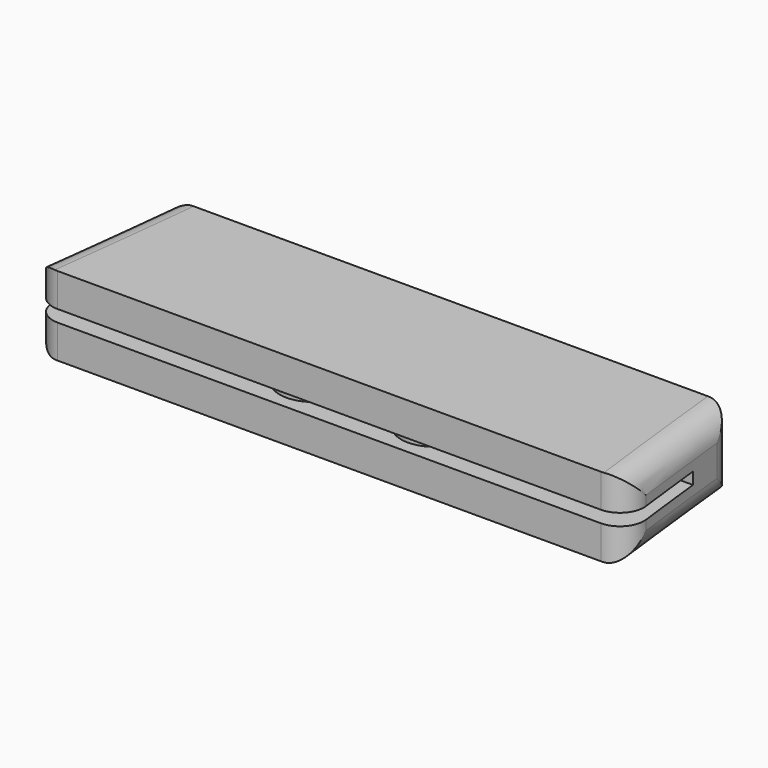
from build123d import *

# Parameters (mm, degrees)
F1_DEPTH = 4.191
F2_W     = 31.75
F2_H     = 0.635
F3_DEPTH = 5.08
F5_DEPTH = 4.191
F6_R     = 1.27


with BuildPart() as f1:
    # F0 (on Top) → F1 (new body)
    with BuildSketch(Plane.XY):
        with BuildLine():
            Line((30.8222222764, 8.072550722), (0.9351527642, 8.072550722))
            ThreePointArc((0.9351527642, 8.072550722), (0.4877546279, 4.0339378418), (0, 0))
            Line((0, 0), (10.9474, 0))
            Line((10.9474, 0), (14.4018, 0))
            Line((14.4018, 0), (17.3482, 0))
            Line((17.3482, 0), (20.8026, 0))
            Line((20.8026, 0), (31.75, 0))
            ThreePointArc((31.75, 0), (31.2660920194, 4.033974565), (30.8222222764, 8.072550722))
        make_face()
    extrude(amount=F1_DEPTH)

    # F2 (on face) → F3 (cut)
    with BuildSketch(Plane.XZ):
        with Locations((15.875, 2.0955)):
            Rectangle(F2_W, F2_H)
    extrude(amount=-F3_DEPTH, mode=Mode.SUBTRACT)

    # F4 (on face) → F5 (join)
    with BuildSketch(Plane.XY.offset(4.191)):
        with BuildLine():
            Line((14.8268397257, 5.08), (11.3216397257, 5.08))
            Line((11.3216397257, 5.08), (11.3216397257, 2.413))
            ThreePointArc((11.3216397257, 2.413), (13.0742397257, 0.6604), (14.8268397257, 2.413))
            Line((14.8268397257, 2.413), (14.8268397257, 5.08))
        make_face()
        with BuildLine():
            Line((21.2784397257, 5.08), (17.7732397257, 5.08))
            Line((17.7732397257, 5.08), (17.7732397257, 2.413))
            ThreePointArc((17.7732397257, 2.413), (19.5258397257, 0.6604), (21.2784397257, 2.413))
            Line((21.2784397257, 2.413), (21.2784397257, 5.08))
        make_face()
    extrude(amount=-F5_DEPTH)

    # F6
    f6_edges = [f1.edges().sort_by_distance(p)[0] for p in [
        (0.935153, 8.072551, 2.0955),
        (30.822222, 8.072551, 2.0955),
        (31.266092, 4.033975, 4.191),
        (0.487755, 4.033938, 4.191),
        (0.487755, 4.033938, 0),
        (31.266092, 4.033975, 0),
        (31.75, 0, 3.302),
        (31.75, 0, 0.889),
        (0, 0, 0.889),
        (0, 0, 3.302),
    ]]
    fillet(f6_edges, radius=F6_R)


solid = f1.part
